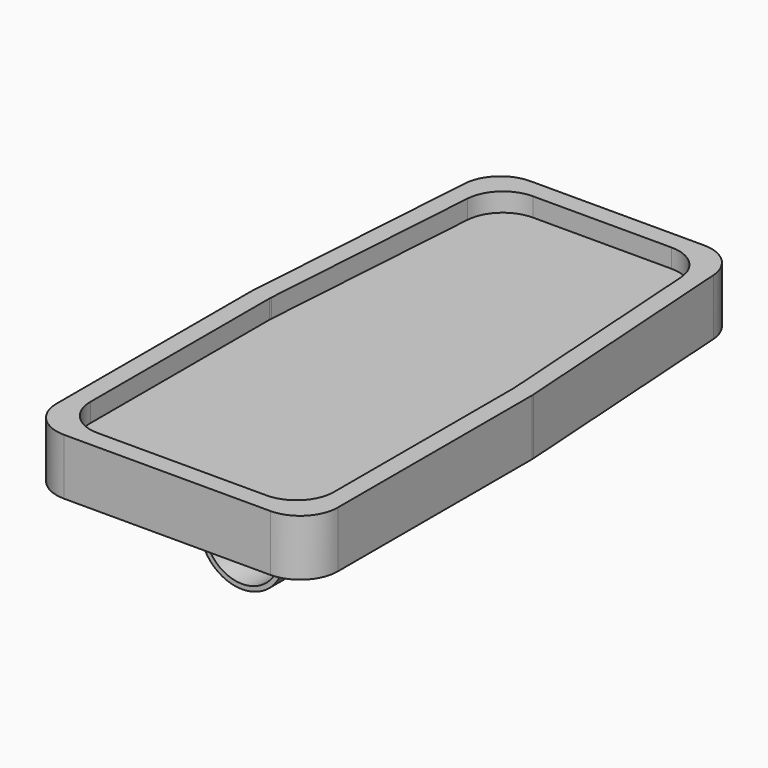
from build123d import *

# Parameters (mm, degrees)
F1_DEPTH    = 30
F2_DEPTH    = 20
F3_T1_DEPTH = 10
F3_T3_DEPTH = 11.6648189186
F3_T5_DEPTH = 130
F3_T7_DEPTH = 123.5553091892
F3_T9_DEPTH = 33.3296378373
F5_W        = 45
F5_H        = 200
F6_DEPTH    = 45
F7_R        = 20
F8_DEPTH    = 200
F9_R        = 22.49999


# Not quite as in the source:
# - a fillet or chamfer that OpenCascade refuses, or shapes differently, is made with other operations: its cross-section is extruded or revolved along the edge and cut away or added
# - two fillets or chamfers of one size are made in one step
# - a fillet or chamfer is up to 0.001 mm smaller than in the source, because OpenCascade refuses the exact size


with BuildPart() as f1:
    # F0 (on Top) → F1 (new body)
    with BuildSketch(Plane.XY):
        Polygon((65, 150), (-65, 150), (-75, 0), (-75, -150), (75, -150), (75, 0), align=None)
        Polygon((-65, 0), (-55.6666666667, 140), (55.6666666667, 140), (65, 0), (65, -140), (-65, -140), align=None, mode=Mode.SUBTRACT)
    extrude(amount=F1_DEPTH)

    # F0 (on Top) → F2 (join)
    with BuildSketch(Plane.XY):
        Polygon((55.6666666667, 140), (-55.6666666667, 140), (-65, 0), (-65, -140), (65, -140), (65, 0), align=None)
    extrude(amount=F2_DEPTH)

    # F3: fillet of radius 20 on 12 edges, made by hand

    # F3_s2 → F3_t1 (join)
    with BuildSketch(Plane.XY.offset(20)):
        with BuildLine():
            ThreePointArc((-56.911307986, 121.3303802105), (-50.6192865397, 134.6049238993), (-36.9556048288, 140))
            Line((-36.9556048288, 140), (-55.6666666667, 140))
            Line((-55.6666666667, 140), (-56.911307986, 121.3303802105))
        make_face()
        with BuildLine():
            ThreePointArc((36.9556048288, 140), (50.6192865397, 134.6049238993), (56.911307986, 121.3303802105))
            Line((56.911307986, 121.3303802105), (55.6666666667, 140))
            Line((55.6666666667, 140), (36.9556048288, 140))
        make_face()
        with BuildLine():
            ThreePointArc((65, -120), (59.1421356237, -134.1421356237), (45, -140))
            Line((45, -140), (65, -140))
            Line((65, -140), (65, -120))
        make_face()
        with BuildLine():
            ThreePointArc((-45, -140), (-59.1421356237, -134.1421356237), (-65, -120))
            Line((-65, -120), (-65, -140))
            Line((-65, -140), (-45, -140))
        make_face()
    extrude(amount=F3_T1_DEPTH)

    # F3_s4 → F3_t3 (join)
    with BuildSketch(Plane.XY.offset(18.3351810814)):
        with BuildLine():
            ThreePointArc((-64.9557031571, 0.664452643), (-64.9889227216, -0.0003688333), (-65, -0.6659275675))
            Line((-65, -0.6659275675), (-65, 0))
            Line((-65, 0), (-64.9557031571, 0.664452643))
        make_face()
        with BuildLine():
            ThreePointArc((64.9557031571, 0.664452643), (64.9889227216, -0.0003688333), (65, -0.6659275675))
            Line((65, -0.6659275675), (65, 0))
            Line((65, 0), (64.9557031571, 0.664452643))
        make_face()
    extrude(amount=F3_T3_DEPTH)

    # F3_s6 → F3_t5 (cut)
    with BuildSketch(Plane.XY.offset(-50)):
        with BuildLine():
            ThreePointArc((75, -130), (69.1421356237, -144.1421356237), (55, -150))
            Line((55, -150), (75, -150))
            Line((75, -150), (75, -130))
        make_face()
        with BuildLine():
            ThreePointArc((-75, -130), (-69.1421356237, -144.1421356237), (-55, -150))
            Line((-55, -150), (-75, -150))
            Line((-75, -150), (-75, -130))
        make_face()
    extrude(amount=F3_T5_DEPTH, mode=Mode.SUBTRACT)

    # F3_s8 → F3_t7 (cut)
    with BuildSketch(Plane.XY.offset(-46.7776545946)):
        with BuildLine():
            ThreePointArc((46.2889381622, 150), (59.952619873, 144.6049238993), (66.2446413193, 131.3303802105))
            Line((66.2446413193, 131.3303802105), (65, 150))
            Line((65, 150), (46.2889381622, 150))
        make_face()
        with BuildLine():
            ThreePointArc((-46.2889381622, 150), (-59.952619873, 144.6049238993), (-66.2446413193, 131.3303802105))
            Line((-66.2446413193, 131.3303802105), (-65, 150))
            Line((-65, 150), (-46.2889381622, 150))
        make_face()
    extrude(amount=F3_T7_DEPTH, mode=Mode.SUBTRACT)

    # F3_s10 → F3_t9 (cut)
    with BuildSketch(Plane.XY.offset(-1.6648189186)):
        with BuildLine():
            ThreePointArc((74.9557031571, 0.664452643), (74.9889227216, -0.0003688333), (75, -0.6659275675))
            Line((75, -0.6659275675), (75, 0))
            Line((75, 0), (74.9557031571, 0.664452643))
        make_face()
        with BuildLine():
            ThreePointArc((-74.9557031571, 0.664452643), (-74.9889227216, -0.0003688333), (-75, -0.6659275675))
            Line((-75, -0.6659275675), (-75, 0))
            Line((-75, 0), (-74.9557031571, 0.664452643))
        make_face()
    extrude(amount=F3_T9_DEPTH, mode=Mode.SUBTRACT)

    # F5 (on face) → F6 (join)
    with BuildSketch(Plane.XY):
        Rectangle(F5_W, F5_H)
    extrude(amount=-F6_DEPTH)

    # F7 (on face) → F8 (cut, through all)
    with BuildSketch(Plane.XZ.offset(100)):
        with Locations((0, -22.5)):
            Circle(F7_R)
    extrude(amount=-F8_DEPTH, mode=Mode.SUBTRACT)

    # F9 (radius 22.5 in the source; OpenCascade refuses exactly that, so slightly less here)
    f9_edges = [f1.edges().sort_by_distance(p)[0] for p in [
        (-22.5, 0, -45),
        (22.5, 0, -45),
    ]]
    fillet(f9_edges, radius=F9_R)


solid = f1.part
